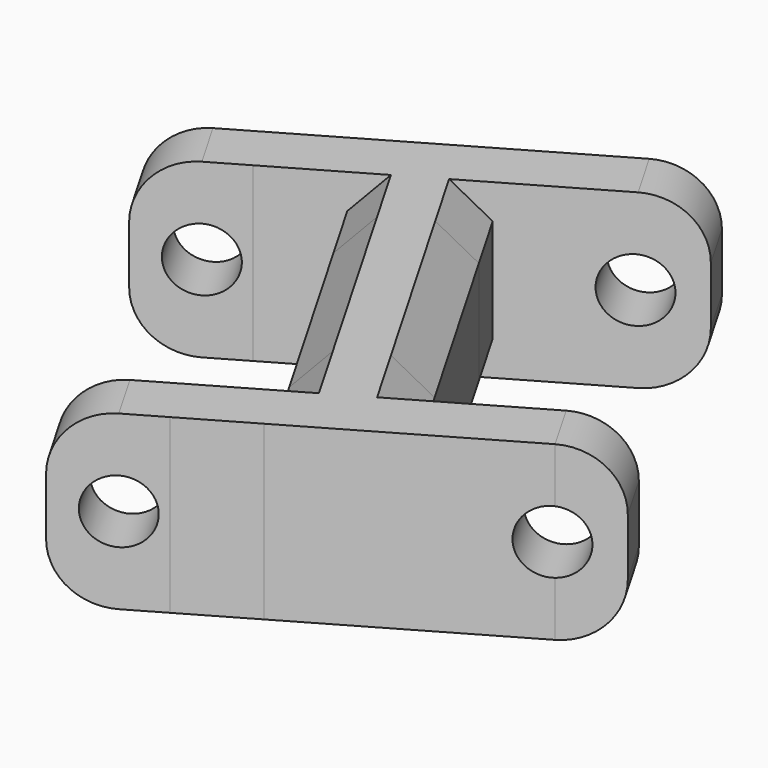
from build123d import *

# Parameters (mm, degrees)
F1_DEPTH = 15
F3_DEPTH = 60
F4_SIZE  = 3
F5_R     = 5


with BuildPart() as f1:
    # F0 (on Top) → F1 (new body)
    with BuildSketch(Plane.XY):
        Polygon((-84.375, 42.2187384345), (-78.75, 45.4663336987), (-61.4294919243, 55.4663336987), (-63.9294919243, 59.7964607176), (-72.5897459622, 54.7964607176), (-75.7147459622, 60.2091194913), (-84.375, 55.2091194913), (-81.25, 49.7964607176), (-86.875, 46.5488654534), align=None)
        Polygon((-61.4294919243, 55.4663336987), (-57.0993649054, 57.9663336987), (-59.5993649054, 62.2964607176), (-63.9294919243, 59.7964607176), align=None)
        Polygon((-91.7403810568, 37.9663336987), (-84.375, 42.2187384345), (-86.875, 46.5488654534), (-94.2403810568, 42.2964607176), align=None)
        Polygon((-84.375, 55.2091194913), (-75.7147459622, 60.2091194913), (-85.7147459622, 77.5296275669), (-87.793790014, 76.329290924), (-94.375, 72.5296275669), align=None)
        Polygon((-87.793790014, 76.329290924), (-85.7147459622, 77.5296275669), (-88.8397459622, 82.9422863406), (-75.8493649054, 90.4422863406), (-78.3493115936, 94.7723526968), (-100, 82.2724133595), (-105.625, 79.0248180953), (-103.125, 74.6946910764), (-97.5, 77.9422863406), (-94.375, 72.5296275669), align=None)
        Polygon((-110.4903810568, 70.4422863406), (-103.125, 74.6946910764), (-105.625, 79.0248180953), (-112.9903810568, 74.7724133595), align=None)
    extrude(amount=F1_DEPTH)

    # F2 (on face) → F3 (cut)
    with BuildSketch(Plane(origin=(-39.375, 68.199500548, 0), x_dir=(0.8660254038, 0.5, 0), z_dir=(0.5, -0.8660254038, 0))):
        with BuildLine():
            ThreePointArc((-52.7163336987, 7.5), (-55.4663336987, 10.25), (-58.2163336987, 7.5))
            Line((-58.2163336987, 7.5), (-55.4663336987, 7.5))
            Line((-55.4663336987, 7.5), (-52.7163336987, 7.5))
        make_face()
        with BuildLine():
            Line((-55.4663336987, 7.5), (-58.2163336987, 7.5))
            ThreePointArc((-58.2163336987, 7.5), (-55.4663336987, 4.75), (-52.7163336987, 7.5))
            Line((-52.7163336987, 7.5), (-55.4663336987, 7.5))
        make_face()
        with BuildLine():
            ThreePointArc((-22.8953336987, 7.5), (-25.6453336987, 10.25), (-28.3953336987, 7.5))
            ThreePointArc((-28.3953336987, 7.5), (-25.6453336987, 4.75), (-22.8953336987, 7.5))
        make_face()
    extrude(amount=-F3_DEPTH, mode=Mode.SUBTRACT)

    # F4
    f4_edges = [f1.edges().sort_by_distance(p)[0] for p in [
        (-89.375, 63.869374, 15),
        (-80.714746, 68.869374, 15),
        (-89.375, 63.869374, 0),
        (-80.714746, 68.869374, 0),
    ]]
    chamfer(f4_edges, length=F4_SIZE)

    # F5
    f5_edges = [f1.edges().sort_by_distance(p)[0] for p in [
        (-92.990381, 40.131397, 0),
        (-111.740381, 72.60735, 0),
        (-111.740381, 72.60735, 15),
        (-92.990381, 40.131397, 15),
        (-58.349365, 60.131397, 15),
        (-58.349365, 60.131397, 0),
        (-77.099338, 92.60732, 15),
        (-77.099338, 92.60732, 0),
    ]]
    fillet(f5_edges, radius=F5_R)


solid = f1.part
